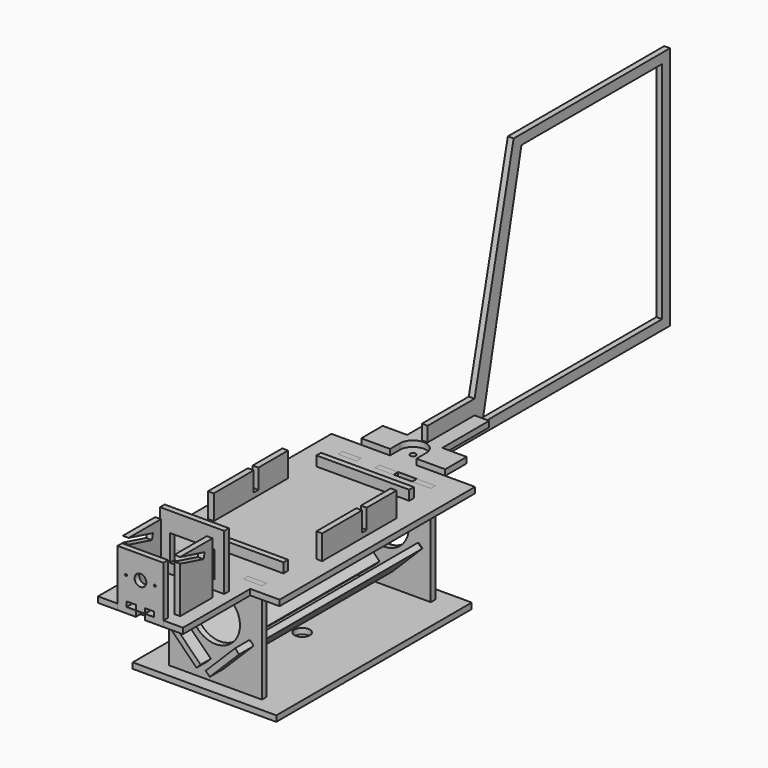
from build123d import *

# Parameters (mm, degrees)
F0_W      = 74.6252
F0_H      = 127
F0_W_2    = 9.652
F0_H_2    = 2.99974
F0_R      = 3.999992
F1_DEPTH  = 2.99974
F2_R      = 12.7
F3_DEPTH  = 2.99974
F4_R      = 12.7
F5_DEPTH  = 2.99974
F7_DEPTH  = 2.99974
F9_DEPTH  = 2.99974
F10_W     = 2.99974
F10_H     = 2.99974
F10_H_2   = 3.02514
F10_W_2   = 4.76504
F10_W_3   = 9.652
F10_H_3   = 9.652
F10_R     = 1.4986
F11_DEPTH = 2.99974
F13_DEPTH = 2.99974
F15_DEPTH = 2.99974
F17_DEPTH = 2.99974
F19_DEPTH = 2.99974
F21_DEPTH = 2.99974
F23_DEPTH = 2.99974
F24_W     = 23.1953308
F24_H     = 13.6850882
F25_DEPTH = 2.99974
F27_DEPTH = 2.99974
F29_DEPTH = 2.99974
F30_R     = 0.508
F30_R_2   = 3.0353
F31_DEPTH = 2.99974


# Not quite as in the source:
# - ends of sketch curves that miss each other by under 0.0002 mm in the source are joined


with BuildPart() as f1:
    # F0 (on Top) → F1 (new body)
    with BuildSketch(Plane.XY):
        with Locations((1.5711590482, -0.3042911887)):
            Rectangle(F0_W, F0_H)
        with Locations((-17.7328409518, -55.1441611887)):
            Rectangle(F0_W_2, F0_H_2, mode=Mode.SUBTRACT)
        with Locations((1.5711590482, -55.1441611887)):
            Rectangle(F0_W_2, F0_H_2, mode=Mode.SUBTRACT)
        Polygon((25.7011082482, -56.6440565887), (16.0491590482, -56.6440311887), (16.0491590482, -53.6442911887), (25.7011590482, -53.6442911887), align=None, mode=Mode.SUBTRACT)
        with Locations((-17.7328409518, 54.5355788113)):
            Rectangle(F0_W_2, F0_H_2, mode=Mode.SUBTRACT)
        with Locations((1.5711590482, -0.3042657887)):
            Circle(F0_R, mode=Mode.SUBTRACT)
        with Locations((1.5711590482, 54.5355788113)):
            Rectangle(F0_W_2, F0_H_2, mode=Mode.SUBTRACT)
        Polygon((25.7011082482, 53.0356834113), (16.0491590482, 53.0357088113), (16.0491590482, 56.0354488113), (25.7011590482, 56.0354488113), align=None, mode=Mode.SUBTRACT)
    extrude(amount=F1_DEPTH)


with BuildPart() as f3:
    # F2 (on face) → F3 (new body)
    with BuildSketch(Plane.XZ.offset(53.6442911887)):
        Polygon((16.0491590482, 0), (25.7011590482, 0), (25.7011590482, 55.0697654), (16.0491590482, 55.0697654), (16.0491590482, 52.0700254), (6.3971590482, 52.0700254), (6.3971590482, 55.0697654), (-3.2548409518, 55.0697654), (-3.2548409518, 52.0700254), (-12.9068409518, 52.0700254), (-12.9068409518, 55.0697654), (-22.5588409518, 55.0697654), (-22.5588409518, 2.99974), (-12.9068409518, 2.99974), (-3.2548409518, 2.99974), (-3.2548409518, 0), (6.3971590482, 0), (6.3971590482, 2.99974), (16.0491590482, 2.99974), align=None)
        Polygon((-0.9688409518, 12.9540254), (-3.0008409518, 10.9220254), (-18.2672823518, 26.1884668), (-16.2352823518, 28.2204668), align=None, mode=Mode.SUBTRACT)
        Polygon((21.4096004482, 26.1884668), (6.1431590482, 10.9220254), (4.1111590482, 12.9540254), (19.3776004482, 28.2204668), align=None, mode=Mode.SUBTRACT)
        with Locations((1.5711590482, 33.2740254)):
            Circle(F2_R, mode=Mode.SUBTRACT)
    extrude(amount=F3_DEPTH)


with BuildPart() as f5:
    # F4 (on face) → F5 (new body)
    with BuildSketch(Plane(origin=(0.0001395685, 53.0357510458, 0), x_dir=(-1, 2.6316e-06, 0), z_dir=(2.6316e-06, 1, 0))):
        Polygon((12.9070313202, 0), (22.5590313202, 0), (22.5590313202, 55.0697654), (12.9070313202, 55.0697654), (12.9070313202, 52.0700254), (3.2550313202, 52.0700254), (3.2550313202, 55.0697654), (-6.3969686798, 55.0697654), (-6.3969686798, 52.0700254), (-16.0489686798, 52.0700254), (-16.0489686798, 55.0697654), (-25.7009686798, 55.0697654), (-25.7009686798, 2.99974), (-16.0490194797, 2.99974), (-6.3969686798, 2.99974), (-6.3969686798, 0), (3.2550313202, 0), (3.2550313202, 2.99974), (12.9070313202, 2.99974), align=None)
        Polygon((-4.1109686798, 12.9540254), (-6.1429686798, 10.9220254), (-21.4094100798, 26.1884668), (-19.3774100798, 28.2204668), align=None, mode=Mode.SUBTRACT)
        Polygon((18.2674727202, 26.1884668), (3.0010313202, 10.9220254), (0.9690313202, 12.9540254), (16.2354727202, 28.2204668), align=None, mode=Mode.SUBTRACT)
        with Locations((-1.5709686798, 33.2740254)):
            Circle(F4_R, mode=Mode.SUBTRACT)
    extrude(amount=F5_DEPTH)


with BuildPart() as f7:
    # F6 (on face) → F7 (new body)
    with BuildSketch(Plane(origin=(3.9604970399, -1.04224e-05, 3.9604970399), x_dir=(0.7071067812, 1.8608e-06, -0.7071067812), z_dir=(0.7071067812, -1.8608e-06, 0.7071067812))):
        Polygon((-9.8450670921, 63.7520362139), (-31.4350670921, 63.7520362139), (-31.4350670921, -63.2479637861), (-9.8450670921, -63.2479637861), (-9.8450670921, 53.0357876861), (-31.4348989189, 53.0358680355), (-31.434887755, 56.0356080355), (-9.8450670921, 56.0355276861), align=None)
    extrude(amount=F7_DEPTH)


with BuildPart() as f9:
    # F8 (on face) → F9 (new body)
    with BuildSketch(Plane(origin=(-2.3895283601, 6.2883e-06, 2.3895283601), x_dir=(0.7071067812, 1.8608e-06, 0.7071067812), z_dir=(-0.7071067812, 1.8608e-06, 0.7071067812))):
        Polygon((33.3221740836, 61.2139214277), (11.7321740836, 61.2139214277), (11.7321740836, -65.7860785723), (33.3221740836, -65.7860785723), (33.3221740836, 53.0356270334), (12.0669704143, 53.0357061375), (12.0669815782, 56.0354461374), (33.3221740836, 56.0353670334), align=None)
    extrude(amount=F9_DEPTH)


with BuildPart() as f11:
    # F10 (on face) → F11 (new body)
    with BuildSketch(Plane.XY.offset(52.0700254)):
        with BuildLine():
            Line((3.9536790482, -105.4145711887), (8.7187190482, -105.4145711887))
            Line((8.7187190482, -105.4145711887), (8.7187190482, -102.4148311887))
            Line((8.7187190482, -102.4148311887), (13.4837590482, -102.4148311887))
            Line((13.4837590482, -102.4148311887), (13.4837590482, -105.4145711887))
            Line((13.4837590482, -105.4145711887), (23.6437590482, -105.4145711887))
            Line((23.6437590482, -105.4145711887), (23.6437590482, -61.6732311887))
            Line((23.6437590482, -61.6732311887), (38.8837590482, -61.6732311887))
            Line((38.8837590482, -61.6732311887), (38.8837590482, 65.3267688113))
            Line((38.8837590482, 65.3267688113), (8.4037590482, 65.3267688113))
            Line((8.4037590482, 65.3267688113), (8.4037590482, 71.6767688113))
            ThreePointArc((8.4037590482, 71.6767688113), (1.5711590482, 78.5093688113), (-5.2614409518, 71.6767688113))
            Line((-5.2614409518, 71.6767688113), (-5.2614409518, 65.3267688113))
            Line((-5.2614409518, 65.3267688113), (-35.7414409518, 65.3267688113))
            Line((-35.7414409518, 65.3267688113), (-35.7414409518, -61.6732311887))
            Line((-35.7414409518, -61.6732311887), (-20.5014409518, -61.6732311887))
            Line((-20.5014409518, -61.6732311887), (-20.5014409518, -105.4145711887))
            Line((-20.5014409518, -105.4145711887), (-10.3414409518, -105.4145711887))
            Line((-10.3414409518, -105.4145711887), (-10.3414409518, -102.4148311887))
            Line((-10.3414409518, -102.4148311887), (-5.5764009518, -102.4148311887))
            Line((-5.5764009518, -102.4148311887), (-5.5764009518, -105.4145711887))
            Line((-5.5764009518, -105.4145711887), (-0.8113609518, -105.4145711887))
            Line((-0.8113609518, -105.4145711887), (-0.8113609518, -102.4148311887))
            Line((-0.8113609518, -102.4148311887), (3.9536790482, -102.4148311887))
            Line((3.9536790482, -102.4148311887), (3.9536790482, -105.4145711887))
        make_face()
        with Locations((-11.8413109518, -96.7544411887)):
            Rectangle(F10_W, F10_H, mode=Mode.SUBTRACT)
        with Locations((-11.8413109518, -90.7422611887)):
            Rectangle(F10_W, F10_H_2, mode=Mode.SUBTRACT)
        with Locations((-11.8413109518, -84.7300811887)):
            Rectangle(F10_W, F10_H, mode=Mode.SUBTRACT)
        with Locations((-11.8413109518, -78.7306011887)):
            Rectangle(F10_W, F10_H, mode=Mode.SUBTRACT)
        with Locations((-12.7239609518, -70.3333611887)):
            Rectangle(F10_W_2, F10_H, mode=Mode.SUBTRACT)
        with Locations((-3.1938809518, -70.3333611887)):
            Rectangle(F10_W_2, F10_H, mode=Mode.SUBTRACT)
        with Locations((-17.7328409518, -55.1441611887)):
            Rectangle(F10_W_3, F10_H, mode=Mode.SUBTRACT)
        with Locations((-17.7328663518, -41.1741611887)):
            Rectangle(F10_W_3, F10_H, mode=Mode.SUBTRACT)
        Polygon((-28.0986317518, -24.4342657887), (-28.0986063518, -14.7822911887), (-25.0988663518, -14.7822911887), (-25.0988663518, -24.4342911887), align=None, mode=Mode.SUBTRACT)
        with Locations((1.5711590482, -55.1441611887)):
            Rectangle(F10_W_3, F10_H, mode=Mode.SUBTRACT)
        with Locations((1.5711336482, -41.1741611887)):
            Rectangle(F10_W_3, F10_H, mode=Mode.SUBTRACT)
        with Locations((14.9836290482, -96.7544411887)):
            Rectangle(F10_W, F10_H, mode=Mode.SUBTRACT)
        with Locations((14.9836290482, -90.7422611887)):
            Rectangle(F10_W, F10_H_2, mode=Mode.SUBTRACT)
        with Locations((14.9836290482, -84.7300811887)):
            Rectangle(F10_W, F10_H, mode=Mode.SUBTRACT)
        with Locations((6.3361990482, -70.3333611887)):
            Rectangle(F10_W_2, F10_H, mode=Mode.SUBTRACT)
        with Locations((14.9836290482, -78.7306011887)):
            Rectangle(F10_W, F10_H, mode=Mode.SUBTRACT)
        with Locations((15.8662790482, -70.3333611887)):
            Rectangle(F10_W_2, F10_H, mode=Mode.SUBTRACT)
        Polygon((25.7011082482, -56.6440565887), (16.0491590482, -56.6440311887), (16.0491590482, -53.6442911887), (25.7011590482, -53.6442911887), align=None, mode=Mode.SUBTRACT)
        Polygon((25.7011082482, -42.6740819887), (16.0491336482, -42.6740311887), (16.0491336482, -39.6742911887), (25.7011336482, -39.6742911887), align=None, mode=Mode.SUBTRACT)
        Polygon((28.2411082482, -24.4342403887), (28.2411590482, -14.7822911887), (31.2408990482, -14.7822911887), (31.2408990482, -24.4342911887), align=None, mode=Mode.SUBTRACT)
        with Locations((-26.5987363518, -0.3042911887)):
            Rectangle(F10_W, F10_H_3, mode=Mode.SUBTRACT)
        with Locations((-26.5987363518, 18.9997088113)):
            Rectangle(F10_W, F10_H_3, mode=Mode.SUBTRACT)
        with Locations((-17.7328409518, 40.5655788113)):
            Rectangle(F10_W_3, F10_H, mode=Mode.SUBTRACT)
        with Locations((-17.7328409518, 54.5355788113)):
            Rectangle(F10_W_3, F10_H, mode=Mode.SUBTRACT)
        with Locations((1.5711590482, 40.5655788113)):
            Rectangle(F10_W_3, F10_H, mode=Mode.SUBTRACT)
        with Locations((29.7410290482, -0.3042911887)):
            Rectangle(F10_W, F10_H_3, mode=Mode.SUBTRACT)
        with Locations((29.7410290482, 18.9997088113)):
            Rectangle(F10_W, F10_H_3, mode=Mode.SUBTRACT)
        Polygon((6.3971590482, 53.0357088113), (-3.2548409518, 53.0357088113), (-3.2548409518, 56.0354488113), (6.3971590482, 56.0354488113), (16.0491161423, 56.0354488114), (25.7011590482, 56.0354488113), (25.7011082482, 53.0356834113), (16.0491590482, 53.0357088113), align=None, mode=Mode.SUBTRACT)
        with Locations((1.5711590482, 71.6767688113)):
            Circle(F10_R, mode=Mode.SUBTRACT)
        Polygon((25.7011082482, 39.0656834113), (16.0491590482, 39.0657088113), (16.0491590482, 42.0654488113), (25.7011590482, 42.0654488113), align=None, mode=Mode.SUBTRACT)
    extrude(amount=F11_DEPTH)


with BuildPart() as f13:
    # F12 (on face) → F13 (new body)
    with BuildSketch(Plane.XY.offset(55.0697654)):
        with BuildLine():
            Line((3.0710290482, 109.7767688113), (3.0710290482, 94.5367688113))
            Line((3.0710290482, 94.5367688113), (0.0712890482, 94.5367688113))
            Line((0.0712890482, 94.5367688113), (0.0712890482, 109.7767688113))
            Line((0.0712890482, 109.7767688113), (-7.5487109518, 109.7767688113))
            Line((-7.5487109518, 109.7767688113), (-7.5487109518, 79.2967688113))
            Line((-7.5487109518, 79.2967688113), (-20.2487109518, 79.2967688113))
            Line((-20.2487109518, 79.2967688113), (-20.2487109518, 65.3267688113))
            Line((-20.2487109518, 65.3267688113), (-5.2614409518, 65.3267688113))
            Line((-5.2614409518, 65.3267688113), (-5.2614409518, 71.6767688113))
            ThreePointArc((-5.2614409518, 71.6767688113), (1.5711590482, 78.5093688113), (8.4037590482, 71.6767688113))
            Line((8.4037590482, 71.6767688113), (8.4037590482, 65.3267688113))
            Line((8.4037590482, 65.3267688113), (23.3910290482, 65.3267688113))
            Line((23.3910290482, 65.3267688113), (23.3910290482, 79.2967688113))
            Line((23.3910290482, 79.2967688113), (10.6910290482, 79.2967688113))
            Line((10.6910290482, 79.2967688113), (10.6910290482, 109.7767688113))
            Line((10.6910290482, 109.7767688113), (3.0710290482, 109.7767688113))
        make_face()
    extrude(amount=F13_DEPTH)


with BuildPart() as f15:
    # F14 (on face) → F15 (new body)
    with BuildSketch(Plane(origin=(3.0710290482, 0, 0), x_dir=(0, -1, 0), z_dir=(-1, 0, 0))):
        Polygon((-135.1767688113, 174.4497654), (-236.7767688113, 174.4497654), (-236.7767688113, 47.4497654), (-79.2967688113, 47.4497654), (-79.2967688113, 55.0697654), (-94.5367688113, 55.0697654), (-109.7767688113, 55.0697654), (-109.7767688113, 58.0695054), (-94.5367688113, 58.0695054), (-79.2967688113, 58.0695054), (-79.2967688113, 65.6895054), (-109.7767688113, 65.6895054), align=None)
        Polygon((-231.6469594113, 52.5295368), (-231.6971752113, 169.3072052), (-140.2567688113, 169.3697654), (-114.8567688113, 52.5297654), align=None, mode=Mode.SUBTRACT)
    extrude(amount=F15_DEPTH)


with BuildPart() as f17:
    # F16 (on face) → F17 (new body)
    with BuildSketch(Plane.XZ.offset(-42.0654488113)):
        Polygon((-22.5588409518, 60.1497654), (-22.5588409518, 52.0700254), (-12.9068409518, 52.0700254), (-12.9068409518, 55.0697654), (-3.2548409518, 55.0697654), (6.3971590482, 55.0697654), (16.0491590482, 55.0697654), (16.0491590482, 52.0700254), (25.7011336482, 52.0699746), (25.7011590482, 55.0697654), (25.7011590482, 60.1497654), align=None)
    extrude(amount=F17_DEPTH)


with BuildPart() as f19:
    # F18 (on face) → F19 (new body)
    with BuildSketch(Plane(origin=(0, -42.6740311887, 0), x_dir=(-1, 0, 0), z_dir=(0, 1, 0))):
        Polygon((-25.7011082482, 60.1497654), (-25.7011082482, 52.0700254), (-16.0491082482, 52.0700254), (-16.0491082482, 55.0697654), (-6.3971082482, 55.0697654), (3.2548663518, 55.0697654), (12.9068917518, 55.0697654), (12.9068917518, 52.0700254), (22.5588663518, 52.0699746), (22.5588917518, 55.0697654), (22.5588917518, 60.1497654), align=None)
    extrude(amount=F19_DEPTH)


with BuildPart() as f21:
    # F20 (on face) → F21 (new body)
    with BuildSketch(Plane(origin=(31.2408990482, 0, 0), x_dir=(0, -1, 0), z_dir=(-1, 0, 0))):
        Polygon((-23.8257088113, 67.7697654), (-23.8257088113, 52.0700254), (-14.1737088113, 52.0700254), (-14.1737088113, 55.0697654), (-4.5217088113, 55.0697654), (5.1302911887, 55.0697654), (14.7822911887, 55.0697654), (14.7822911887, 52.0700254), (24.4342657887, 52.0699746), (24.4342911887, 55.0697654), (24.4342911887, 67.7697654), (-1.5219688113, 67.7697654), (-1.5219688113, 57.6097654), (-4.5217088113, 57.6097654), (-4.5217088113, 67.7697654), align=None)
    extrude(amount=F21_DEPTH)


with BuildPart() as f23:
    # F22 (on face) → F23 (new body)
    with BuildSketch(Plane(origin=(-25.0988663518, 0, 0), x_dir=(0, -1, 0), z_dir=(-1, 0, 0))):
        Polygon((-23.8257088113, 67.7697654), (-23.8257088113, 52.0700254), (-14.1737088113, 52.0700254), (-14.1737088113, 55.0697654), (-4.5217088113, 55.0697654), (5.1302911887, 55.0697654), (14.7822911887, 55.0697654), (14.7822911887, 52.0700254), (24.4342657887, 52.0699746), (24.4342911887, 55.0697654), (24.4342911887, 67.7697654), (-1.5219688113, 67.7697654), (-1.5219688113, 57.6097654), (-4.5217088113, 57.6097654), (-4.5217088113, 67.7697654), align=None)
    extrude(amount=F23_DEPTH)


with BuildPart() as f25:
    # F24 (on face) → F25 (new body)
    with BuildSketch(Plane.XZ.offset(68.8334911887)):
        Polygon((3.9536790482, 52.0700254), (8.7187190482, 52.0700254), (8.7187190482, 55.0697654), (13.4837590482, 55.0697654), (13.4837590482, 52.0700254), (18.2487990482, 52.0700254), (18.2487990482, 83.9749654), (-15.1064809518, 83.9749654), (-15.1064809518, 52.0700254), (-10.3414409518, 52.0700254), (-10.3414409518, 55.0697654), (-5.5764009518, 55.0697654), (-0.8113609518, 55.0697654), (3.9536790482, 55.0697654), align=None)
        with Locations((1.5711336482, 66.9923095)):
            Rectangle(F24_W, F24_H, mode=Mode.SUBTRACT)
    extrude(amount=F25_DEPTH)


with BuildPart() as f27:
    # F26 (on face) → F27 (new body)
    with BuildSketch(Plane.YZ.offset(-13.3411809518)):
        Polygon((-83.2302111887, 52.0700254), (-83.2302111887, 55.0697654), (-80.2304711887, 55.0697654), (-80.2304711887, 52.0700254), (-77.2307311887, 52.0700254), (-77.2307311887, 82.2018168), (-98.2543111887, 82.2018168), (-82.3107311887, 77.9297654), (-83.0871329887, 75.032235), (-98.2543111887, 79.0962604), (-98.2543111887, 52.0700254), (-95.2545711887, 52.0700254), (-95.2545711887, 55.0697654), (-92.2548311887, 55.0697654), (-89.2550911887, 55.0697654), (-89.2296911887, 55.0697654), (-86.2553511887, 55.0697654), (-86.2553511887, 52.0700254), align=None)
    extrude(amount=F27_DEPTH)


with BuildPart() as f29:
    # F28 (on face) → F29 (new body)
    with BuildSketch(Plane.YZ.offset(13.4837590482)):
        Polygon((-83.2302111887, 52.0700254), (-83.2302111887, 55.0697654), (-80.2304711887, 55.0697654), (-80.2304711887, 52.0700254), (-77.2307311887, 52.0700254), (-77.2307311887, 82.2018168), (-98.2543111887, 82.2018168), (-82.3107311887, 77.9297654), (-83.0871329887, 75.032235), (-98.2543111887, 79.0962604), (-98.2543111887, 52.0700254), (-95.2545711887, 52.0700254), (-95.2545711887, 55.0697654), (-92.2548311887, 55.0697654), (-89.2550911887, 55.0697654), (-89.2296911887, 55.0697654), (-86.2553511887, 55.0697654), (-86.2553511887, 52.0700254), align=None)
    extrude(amount=F29_DEPTH)


with BuildPart() as f31:
    # F30 (on face) → F31 (new body)
    with BuildSketch(Plane.XZ.offset(102.4148311887)):
        Polygon((13.4837590482, 52.0700254), (13.4837590482, 81.4705254), (-10.3414409518, 81.4705254), (-10.3414409518, 52.0700254), (-0.8113609518, 52.0700254), (-0.8113609518, 54.6100254), (-5.5764009518, 54.6100254), (-5.5764009518, 57.6097654), (-0.8113609518, 57.6097654), (-0.8113609518, 55.0697654), (3.9536790482, 55.0697654), (3.9536790482, 57.6097654), (8.7187190482, 57.6097654), (8.7187190482, 54.6100254), (3.9536790482, 54.6100254), (3.9536790482, 52.0700254), align=None)
        with Locations((-5.9027909518, 69.5579254)):
            Circle(F30_R, mode=Mode.SUBTRACT)
        with Locations((1.5711590482, 69.5579254)):
            Circle(F30_R_2, mode=Mode.SUBTRACT)
        with Locations((9.0451090482, 69.5579254)):
            Circle(F30_R, mode=Mode.SUBTRACT)
    extrude(amount=F31_DEPTH)


solid = Compound([f1.part, f3.part, f5.part, f7.part, f9.part, f11.part, f13.part, f15.part, f17.part, f19.part, f21.part, f23.part, f25.part, f27.part, f29.part, f31.part])
